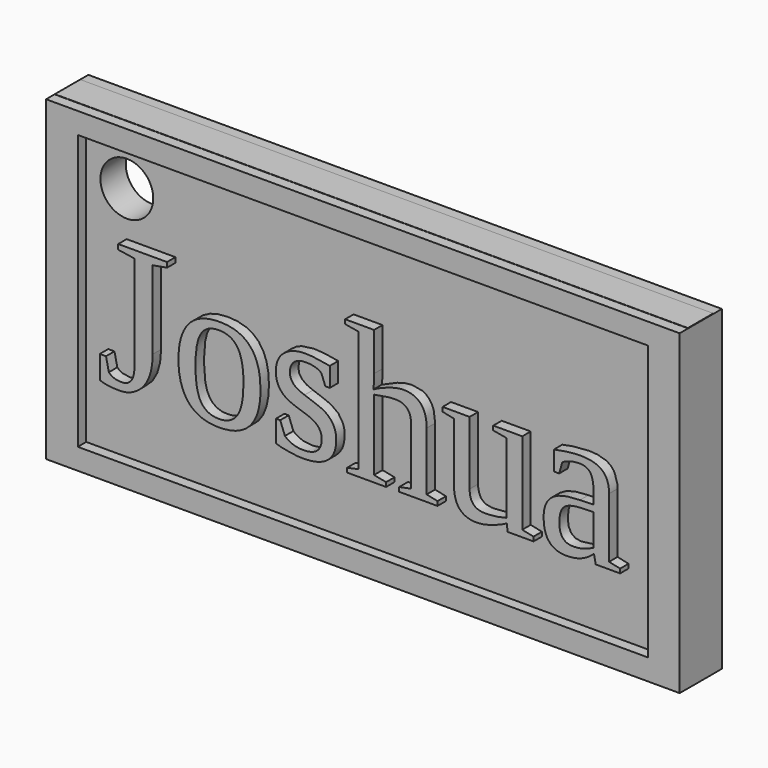
from build123d import *

# Parameters (mm, degrees)
F0_W         = 76.2
F0_H         = 38.1
F0_W_2       = 68.58
F0_H_2       = 33.02
F2_DEPTH     = 3.175
F1_TEXT_SIZE = 23.2833333333
F3_DEPTH     = 3.175
F4_W         = 76.1385411024
F4_H         = 38.1614528596
F5_DEPTH     = 1.905
F7_D         = 6.35


# Not quite as in the source:
# - Text() gives the source's letters only with a copy of the font that has no kerning and outlines rounded to 1/6400 em; it was checked with that copy


with BuildPart() as f2:
    # F0 (on Front) → F2 (new body, symmetric)
    with BuildSketch(Plane.XZ):
        Rectangle(F0_W, F0_H)
        Rectangle(F0_W_2, F0_H_2, mode=Mode.SUBTRACT)
    extrude(amount=F2_DEPTH, both=True)


with BuildPart() as f3:
    # F1 (on Front) → F3 (new body, symmetric)
    with BuildSketch(Plane.XZ):
        with Locations((-32.1298592921, -8.7032554925)):
            Text('Joshua', F1_TEXT_SIZE, font='Tinos', text_align=(TextAlign.LEFT, TextAlign.BOTTOM))
    extrude(amount=F3_DEPTH, both=True)


with BuildPart() as f5:
    # F4 (on face) → F5 (new body, symmetric)
    with BuildSketch(Plane.XZ):
        Rectangle(F4_W, F4_H)
    extrude(amount=F5_DEPTH, both=True)

    # F7 (through all)
    with Locations(Plane.XZ.offset(3.175)):
        with Locations((-29.4045973569, 11.8908863515)):
            Hole(F7_D / 2)


solid = Compound([f2.part, f3.part, f5.part])
